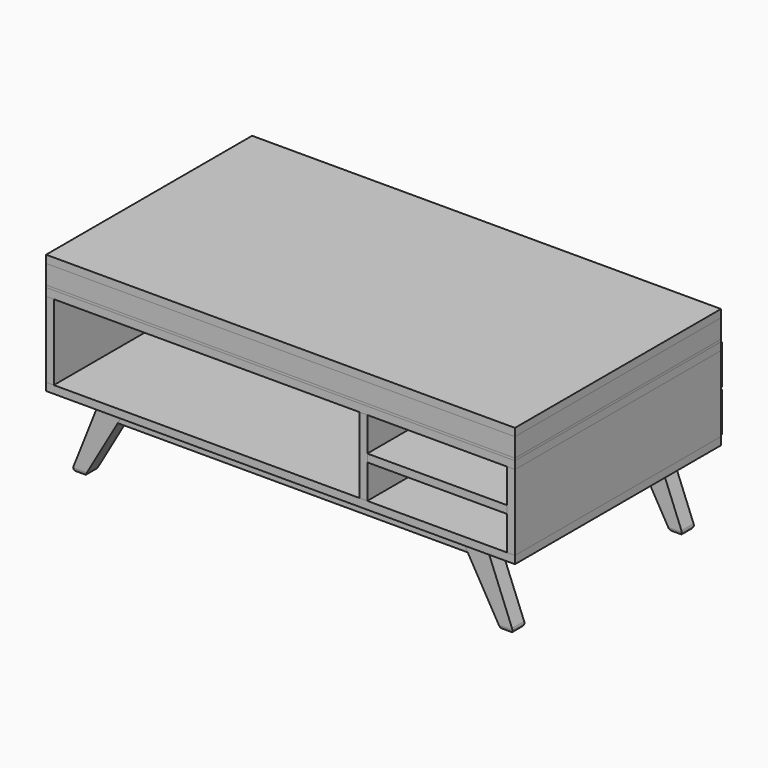
from build123d import *

# Parameters (mm, degrees)
F1_DEPTH       = 340.5
F1_DEPTH_BACK  = 340.5
F2_DEPTH       = 340.5
F2_DEPTH_BACK  = 340.5
F0_W           = 20.5
F0_H           = 200
F3_DEPTH       = 340.5
F3_DEPTH_BACK  = 340.5
F6_DEPTH       = 40
F7_R           = 10
F7_2_R         = 10
F8_DEPTH       = 40
F10_W          = 46.1880215352
F10_H          = 40
F11_DEPTH      = 520
F12_W          = 7
F12_H          = 96.75
F13_DEPTH      = 20
F14_W          = 1240
F14_H          = 681
F14_W_2        = 1230
F14_H_2        = 671
F14_W_3        = 1199
F14_H_3        = 640
F15_DEPTH      = 6
F16_W          = 898.5
F16_H          = 637
F17_DEPTH      = 3
F16_W_2        = 297.5
F18_DEPTH      = 3
F19_DEPTH      = 50
F20_W          = 1240
F20_H          = 681
F21_DEPTH      = 20.5
F23_DEPTH      = 370
F0_W_2         = 370
F0_H_2         = 20.5
F24_DEPTH      = 19.5
F24_DEPTH_BACK = 340.5


# Not quite as in the source:
# - a feature names something its author has since deleted; it is built from what else it names


with BuildPart() as f1:
    # F0 (on Front) → F1 (new body, two sides)
    with BuildSketch(Plane.XZ) as f1_sk:
        Polygon((-599.5, -220.5), (-620, -220.5), (-620, -241), (620, -241), (620, -220.5), (599.5, -220.5), (229.5, -220.5), (209, -220.5), align=None)
    extrude(amount=F1_DEPTH)
    extrude(f1_sk.sketch, amount=-F1_DEPTH_BACK)


with BuildPart() as f2:
    # F0 (on Front) → F2 (new body, two sides)
    with BuildSketch(Plane.XZ) as f2_sk:
        Polygon((229.5, -20.5), (209, -20.5), (209, -220.5), (229.5, -220.5), (229.5, -130.75), (229.5, -110.25), align=None)
    extrude(amount=F2_DEPTH)
    extrude(f2_sk.sketch, amount=-F2_DEPTH_BACK)


with BuildPart() as f2b:
    # F0 (on Front) → F2, piece 2 (new body, two sides)
    with BuildSketch(Plane.XZ) as f2_2_sk:
        with Locations((-609.75, -120.5)):
            Rectangle(F0_W, F0_H)
    extrude(amount=F2_DEPTH)
    extrude(f2_2_sk.sketch, amount=-F2_DEPTH_BACK)


with BuildPart() as f2c:
    # F0 (on Front) → F2, piece 3 (new body, two sides)
    with BuildSketch(Plane.XZ) as f2_3_sk:
        Polygon((620, -220.5), (620, -20.5), (599.5, -20.5), (599.5, -110.25), (599.5, -130.75), (599.5, -220.5), align=None)
    extrude(amount=F2_DEPTH)
    extrude(f2_3_sk.sketch, amount=-F2_DEPTH_BACK)


with BuildPart() as f3:
    # F0 (on Front) → F3 (new body, two sides)
    with BuildSketch(Plane.XZ) as f3_sk:
        Polygon((620, 0), (-620, 0), (-620, -20.5), (-599.5, -20.5), (209, -20.5), (229.5, -20.5), (599.5, -20.5), (620, -20.5), align=None)
    extrude(amount=F3_DEPTH)
    extrude(f3_sk.sketch, amount=-F3_DEPTH_BACK)


with BuildPart() as f6:
    # F5 (on offset) → F6 (new body)
    with BuildSketch(Plane.XZ.offset(260)):
        Polygon((-439.5780408782, -241), (-508.860073181, -241), (-585.3589838486, -433.5), (-550.7179676972, -433.5), (-462.6720516458, -281), align=None)
    extrude(amount=F6_DEPTH)

    # F7
    f7_edges = [f6.edges().sort_by_distance(p)[0] for p in [
        (-568.038476, -300, -433.5),
        (-550.717968, -280, -433.5),
        (-568.038476, -260, -433.5),
        (-585.358984, -280, -433.5),
    ]]
    fillet(f7_edges, radius=F7_R)


with BuildPart() as f6b:
    # F5 (on offset) → F6, piece 2 (new body)
    with BuildSketch(Plane.XZ.offset(260)):
        Polygon((508.860073181, -241), (439.5780408782, -241), (462.6720516458, -281), (550.7179676972, -433.5), (585.3589838486, -433.5), align=None)
    extrude(amount=F6_DEPTH)

    # F7#2
    f7_2_edges = [f6b.edges().sort_by_distance(p)[0] for p in [
        (568.038476, -300, -433.5),
        (550.717968, -280, -433.5),
        (568.038476, -260, -433.5),
        (585.358984, -280, -433.5),
    ]]
    fillet(f7_2_edges, radius=F7_2_R)


with BuildPart() as f8:
    # F5 (on offset) → F8 (new body)
    with BuildSketch(Plane.XZ.offset(260)):
        Polygon((439.5780408782, -241), (-439.5780408782, -241), (-462.6720516458, -281), (462.6720516458, -281), align=None)
    extrude(amount=F8_DEPTH)


with BuildPart() as f9_1:
    # F9: instance of F6
    add(f6.part.mirror(Plane.XZ))


with BuildPart() as f9_2:
    # F9: instance of F6b
    add(f6b.part.mirror(Plane.XZ))


with BuildPart() as f9_3:
    # F9: instance of F8
    add(f8.part.mirror(Plane.XZ))


with BuildPart() as f11:
    # F10 (on face) → F11 (new body, through all)
    with BuildSketch(Plane.XZ.offset(260)):
        with Locations((485.7660624134, -261)):
            Rectangle(F10_W, F10_H)
    extrude(amount=-F11_DEPTH)


with BuildPart() as f11b:
    # F10 (on face) → F11, piece 2 (new body, through all)
    with BuildSketch(Plane.XZ.offset(260)):
        with Locations((-485.7660624134, -261)):
            Rectangle(F10_W, F10_H)
    extrude(amount=-F11_DEPTH)


with BuildPart() as f13:
    # F12 (on face) → F13 (new body)
    with BuildSketch(Plane(origin=(0, 340.5, 0), x_dir=(-1, 0, 0), z_dir=(0, 1, 0))):
        with Locations((-603, -68.875)):
            Rectangle(F12_W, F12_H)
        Polygon((-222.5, -117.25), (-222.5, -13.5), (-606.5, -13.5), (-606.5, -20.5), (-599.5, -20.5), (-599.5, -117.25), align=None)
    extrude(amount=F13_DEPTH)


with BuildPart() as f13b:
    # F12 (on face) → F13, piece 2 (new body)
    with BuildSketch(Plane(origin=(0, 340.5, 0), x_dir=(-1, 0, 0), z_dir=(0, 1, 0))):
        with Locations((-603, -172.125)):
            Rectangle(F12_W, F12_H)
        Polygon((-222.5, -123.75), (-599.5, -123.75), (-599.5, -220.5), (-606.5, -220.5), (-606.5, -227.5), (-222.5, -227.5), align=None)
    extrude(amount=F13_DEPTH)


with BuildPart() as f15:
    # F14 (on face) → F15 (new body)
    with BuildSketch(Plane.XY):
        Rectangle(F14_W, F14_H)
        Rectangle(F14_W_2, F14_H_2, mode=Mode.SUBTRACT)
        Rectangle(F14_W_2, F14_H_2)
        Rectangle(F14_W_3, F14_H_3, mode=Mode.SUBTRACT)
    extrude(amount=F15_DEPTH)


with BuildPart() as f17:
    # F16 (on face) → F17 (new body)
    with BuildSketch(Plane.XY):
        with Locations((-148.75, 0)):
            Rectangle(F16_W, F16_H)
    extrude(amount=F17_DEPTH)


with BuildPart() as f18:
    # F16 (on face) → F18 (new body, through all)
    with BuildSketch(Plane.XY):
        with Locations((449.25, 0)):
            Rectangle(F16_W_2, F16_H)
    extrude(amount=F18_DEPTH)


with BuildPart() as f19:
    # F19 (new): a face of the model
    f19_faces = [f15.part.faces().sort_by_distance(p)[0] for p in [
        (-613.646946667, 0, 6),
    ]]
    extrude(f19_faces, amount=F19_DEPTH)


with BuildPart() as f21:
    # F20 (on face) → F21 (new body)
    with BuildSketch(Plane.XY.offset(56)):
        Rectangle(F20_W, F20_H)
    extrude(amount=F21_DEPTH)


with BuildPart() as f23:
    # F22 (on face) → F23 (new body, through all)
    with BuildSketch(Plane.YZ.offset(229.5)):
        Polygon((40, -20.5), (19.5, -20.5), (19.5, -130.75), (19.5, -220.5), (40, -220.5), (40, -130.75), align=None)
    extrude(amount=F23_DEPTH)


with BuildPart() as f24:
    # F0 (on Front) → F24 (new body, two sides)
    with BuildSketch(Plane.XZ) as f24_sk:
        with Locations((414.5, -120.5)):
            Rectangle(F0_W_2, F0_H_2)
    extrude(amount=-F24_DEPTH)
    extrude(f24_sk.sketch, amount=F24_DEPTH_BACK)


solid = Compound([f1.part, f2.part, f2b.part, f2c.part, f3.part, f6.part, f6b.part, f8.part, f9_1.part, f9_2.part, f9_3.part, f11.part, f11b.part, f13.part, f13b.part, f15.part, f17.part, f18.part, f19.part, f21.part, f23.part, f24.part])
